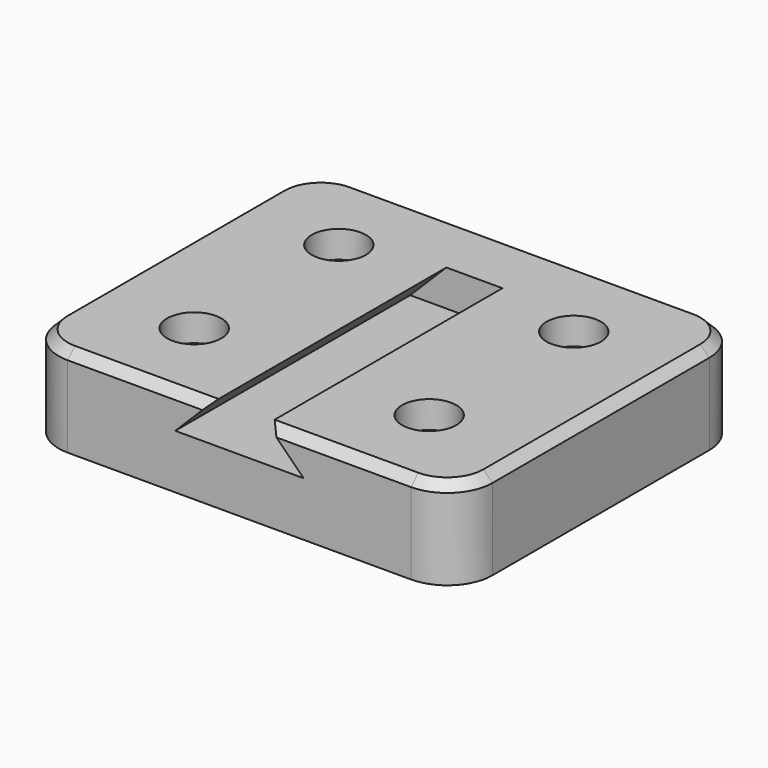
from build123d import *

# Parameters (mm, degrees)
F1_DEPTH       = 20
F2_R           = 5
F5_D           = 3.2
F5_CBORE_D     = 6
F5_CBORE_DEPTH = 3
F6_W           = 18
F6_H           = 7.5
F7_DEPTH       = 10
F8_SIZE        = 1


# Not quite as in the source:
# - a feature of the source that left no trace in its solid (it failed there, or was rolled back) is left out


with BuildPart() as f1:
    # F0 (on Front) → F1 (new body, symmetric)
    with BuildSketch(Plane.XZ):
        Polygon((-24, 4), (-24, 0), (-24, -6), (24, -6), (24, 0), (24, 4), (3.1, 4), (7.1, 0), (-7.1, 0), (-3.1, 4), align=None)
    extrude(amount=F1_DEPTH, both=True)

    # F2
    f2_edges = [f1.edges().sort_by_distance(p)[0] for p in [
        (-24, 20, -1),
        (24, 20, -1),
        (24, -20, -1),
        (-24, -20, -1),
    ]]
    fillet(f2_edges, radius=F2_R)

    # F5 (through all)
    with Locations(Plane.XY.offset(4)):
        with Locations((13, -10), (-13, -10), (13, 10), (-13, 10)):
            CounterBoreHole(F5_D / 2, F5_CBORE_D / 2, F5_CBORE_DEPTH)

    # F6 (on face) → F7 (join)
    with BuildSketch(Plane(origin=(0, 0, -6), x_dir=(1, 0, 0), z_dir=(0, 0, -1))):
        with Locations((0, -16.25)):
            Rectangle(F6_W, F6_H)
    extrude(amount=-F7_DEPTH)

    # F8
    f8_edges = [f1.edges().sort_by_distance(p)[0] for p in [
        (0, 20, 4),
        (-22.535534, 18.535534, 4),
        (-24, 0, 4),
        (-22.535534, -18.535534, 4),
        (-11.05, -20, 4),
        (11.05, -20, 4),
        (22.535534, -18.535534, 4),
        (24, 0, 4),
        (22.535534, 18.535534, 4),
    ]]
    chamfer(f8_edges, length=F8_SIZE)


solid = f1.part
